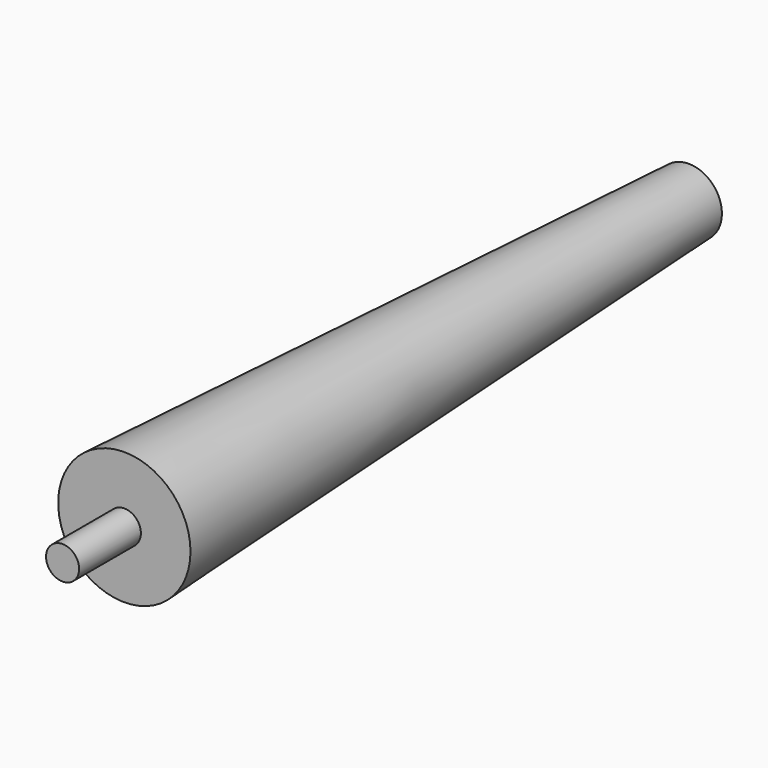
from build123d import *

# Parameters (mm, degrees)
F0_R     = 9.525
F2_R     = 19.05
F4_R     = 4.7625
F5_DEPTH = 22.225


# Not quite as in the source:
# - a feature of the source that left no trace in its solid (it failed there, or was rolled back) is left out


with BuildPart() as f3:
    # F0 (on Front) → F3 section 0
    with BuildSketch(Plane.XZ):
        Circle(F0_R)
    # F2 (on offset) → F3 section 1
    with BuildSketch(Plane.XZ.offset(203.2)):
        Circle(F2_R)
    loft()

    # F4 (on offset) → F5 (join)
    with BuildSketch(Plane.XZ.offset(203.2)):
        Circle(F4_R)
    extrude(amount=F5_DEPTH)


solid = f3.part
